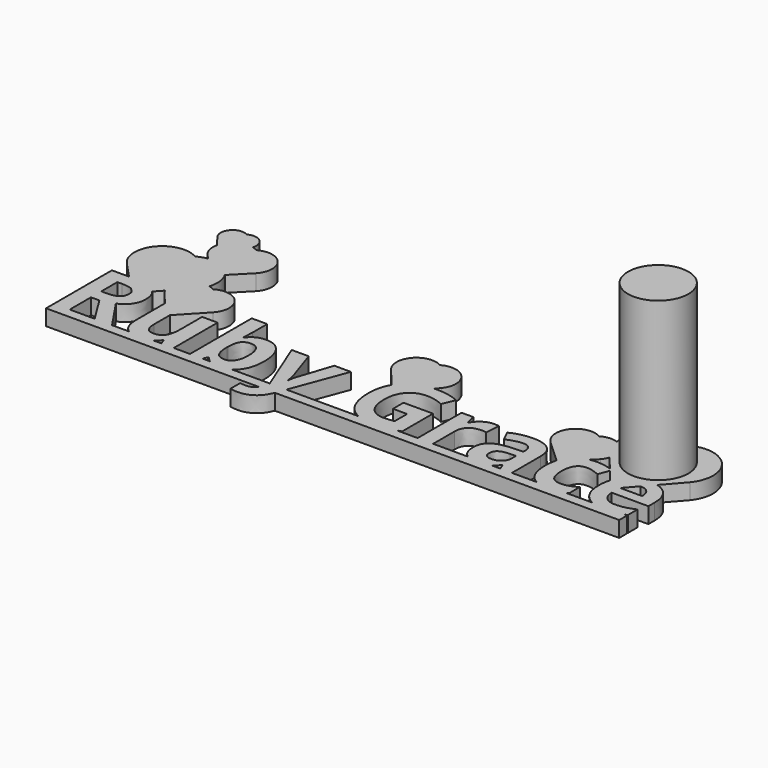
from build123d import *

# Parameters (mm, degrees)
F0_TEXT_SIZE = 13.1857264511
F1_DEPTH     = 2
F2_W         = 72.5544597973
F2_H         = 1.25
F3_DEPTH     = 2
F5_DEPTH     = 2
F6_R         = 3.8242127304
F7_DEPTH     = 20


# Not quite as in the source:
# - a feature names something its author has since deleted; it is built from what else it names
# - Text() gives the source's letters only with a copy of the font that has no kerning and outlines rounded to 1/6400 em; it was checked with that copy


with BuildPart() as f1:
    # F0 (on Top) → F1 (new body)
    with BuildSketch(Plane.XY):
        with Locations((-37.5, -20.9367564448)):
            Text('Ruby Grace', F0_TEXT_SIZE, font='Open Sans', font_style=FontStyle.BOLD, text_align=(TextAlign.LEFT, TextAlign.BOTTOM))
    extrude(amount=F1_DEPTH)

    # F2 (on Top) → F3 (join)
    with BuildSketch(Plane.XY):
        with Locations((-0.0381149905, -21.3117564448)):
            Rectangle(F2_W, F2_H)
    extrude(amount=F3_DEPTH)

    # F4 (on Top) → F5 (join)
    with BuildSketch(Plane.XY):
        with BuildLine():
            ThreePointArc((-22.891365132, -12.3130714182), (-22.7523432909, -9.0480865955), (-25.9622662377, -8.4350224555))
            ThreePointArc((-25.9622662377, -8.4350224555), (-26.2981556025, -8.2731992581), (-26.6543760183, -8.1631291531))
            ThreePointArc((-26.6543760183, -8.1631291531), (-26.7985781504, -8.5405421894), (-26.9853136504, -8.8988223982))
            Line((-26.9853136504, -8.8988223982), (-29.4910691911, -11.6282187871))
            ThreePointArc((-29.4910691911, -11.6282187871), (-29.3216006579, -11.9419906948), (-29.1092122674, -12.2284580847))
            Line((-29.1092122674, -12.2284580847), (-26.104554534, -15.7286860049))
            Line((-26.104554534, -15.7286860049), (-22.891365132, -12.3130714182))
        make_face()
        with BuildLine():
            ThreePointArc((-26.9853136504, -8.8988223982), (-26.7985781504, -8.5405421894), (-26.6543760183, -8.1631291531))
            ThreePointArc((-26.6543760183, -8.1631291531), (-29.1467162118, -9.0164498648), (-29.4910691911, -11.6282187871))
            Line((-29.4910691911, -11.6282187871), (-26.9853136504, -8.8988223982))
        make_face()
        with BuildLine():
            ThreePointArc((-29.4910691911, -11.6282187871), (-29.1467162118, -9.0164498648), (-26.6543760183, -8.1631291531))
            ThreePointArc((-26.6543760183, -8.1631291531), (-26.5125159117, -6.7128085907), (-26.9735699478, -5.3304254314))
            Line((-26.9735699478, -5.3304254314), (-27.8705461931, -6.2434591072))
            Line((-27.8705461931, -6.2434591072), (-30.435701563, -3.633144129))
            ThreePointArc((-30.435701563, -3.633144129), (-31.1099811744, -3.7885760494), (-31.740504166, -4.0736248755))
            ThreePointArc((-31.740504166, -4.0736248755), (-36.233754687, -4.9311026842), (-36.0411839329, -9.5013854919))
            Line((-36.0411839329, -9.5013854919), (-31.7405052483, -14.0784189571))
            Line((-31.7405052483, -14.0784189571), (-29.4910691911, -11.6282187871))
        make_face()
        with BuildLine():
            ThreePointArc((-27.8705461931, -4.3197954554), (-27.3728222762, -4.7814116229), (-26.9735699478, -5.3304254314))
            Line((-26.9735699478, -5.3304254314), (-24.7982677336, -3.1161815346))
            ThreePointArc((-24.7982677336, -3.1161815346), (-24.6612476873, 0.1481262242), (-27.8705463616, 0.7604020253))
            ThreePointArc((-27.8705463616, 0.7604020253), (-28.1874425503, 0.9146740113), (-28.5228848144, 1.0228476104))
            ThreePointArc((-28.5228848144, 1.0228476104), (-28.6581354096, 0.7251189675), (-28.8546919313, 0.4637751287))
            Line((-28.8546919313, 0.4637751287), (-30.8609493077, -1.7959213583))
            Line((-30.8609493077, -1.7959213583), (-31.5607878634, -0.8613195248))
            ThreePointArc((-31.5607878634, -0.8613195248), (-31.5240164461, -2.0926519469), (-30.9036702721, -3.1569368221))
            Line((-30.9036702721, -3.1569368221), (-30.435701563, -3.633144129))
            ThreePointArc((-30.435701563, -3.633144129), (-29.0854748233, -3.7237500646), (-27.8705461931, -4.3197954554))
        make_face()
        with BuildLine():
            Line((-27.8705461931, -6.2434591072), (-26.9735699478, -5.3304254314))
            ThreePointArc((-26.9735699478, -5.3304254314), (-27.3728222762, -4.7814116229), (-27.8705461931, -4.3197954554))
            Line((-27.8705461931, -4.3197954554), (-27.8705461931, -6.2434591072))
        make_face()
        with BuildLine():
            Line((-30.435701563, -3.633144129), (-27.8705461931, -6.2434591072))
            Line((-27.8705461931, -6.2434591072), (-27.8705461931, -4.3197954554))
            ThreePointArc((-27.8705461931, -4.3197954554), (-29.0854748233, -3.7237500646), (-30.435701563, -3.633144129))
        make_face()
        with BuildLine():
            ThreePointArc((-28.8546919313, 0.4637751287), (-28.6581354096, 0.7251189675), (-28.5228848144, 1.0228476104))
            ThreePointArc((-28.5228848144, 1.0228476104), (-30.4382324156, 0.7198861396), (-31.5607878634, -0.8613195248))
            Line((-31.5607878634, -0.8613195248), (-30.8609493077, -1.7959213583))
            Line((-30.8609493077, -1.7959213583), (-28.8546919313, 0.4637751287))
        make_face()
        with BuildLine():
            ThreePointArc((-31.5607878634, -0.8613195248), (-30.4382324156, 0.7198861396), (-28.5228848144, 1.0228476104))
            ThreePointArc((-28.5228848144, 1.0228476104), (-29.002319592, 2.6549750089), (-30.6980615002, 2.7897226685))
            ThreePointArc((-30.6980615002, 2.7897226685), (-32.5699864004, 2.4863172854), (-32.6487473798, 0.5915997956))
            Line((-32.6487473798, 0.5915997956), (-31.5607878634, -0.8613195248))
        make_face()
        with BuildLine():
            ThreePointArc((25.5595961233, -8.9808114981), (24.49969202, -8.8507651041), (23.4822108361, -9.1748651088))
            ThreePointArc((23.4822108361, -9.1748651088), (20.2176636686, -9.8595233663), (20.5393408896, -13.1795457915))
            Line((20.5393408896, -13.1795457915), (23.5436121002, -15.944164712))
            Line((23.5436121002, -15.944164712), (26.6639844478, -12.9268283356))
            ThreePointArc((26.6639844478, -12.9268283356), (26.9346729611, -12.5227898054), (27.1220134693, -12.0739881353))
            Line((27.1220134693, -12.0739881353), (26.4608970103, -11.2691941614))
            ThreePointArc((26.4608970103, -11.2691941614), (25.8299996249, -10.1959947714), (25.5595961233, -8.9808114981))
        make_face()
        with BuildLine():
            ThreePointArc((31.551734789, -5.2660529984), (27.444126715, -5.3304504784), (25.5595961233, -8.9808114981))
            ThreePointArc((25.5595961233, -8.9808114981), (26.9636923968, -10.2127684503), (27.1220134693, -12.0739881353))
            Line((27.1220134693, -12.0739881353), (31.3805904387, -17.2580627952))
            Line((31.3805904387, -17.2580627952), (36.6425725677, -11.2691941614))
            ThreePointArc((36.6425725677, -11.2691941614), (36.6024572806, -6.1430534792), (31.551734789, -5.2660529984))
        make_face()
        with BuildLine():
            ThreePointArc((27.1220134693, -12.0739881353), (26.9636923968, -10.2127684503), (25.5595961233, -8.9808114981))
            ThreePointArc((25.5595961233, -8.9808114981), (25.8299996249, -10.1959947714), (26.4608970103, -11.2691941614))
            Line((26.4608970103, -11.2691941614), (27.1220134693, -12.0739881353))
        make_face()
        with BuildLine():
            ThreePointArc((4.8622423229, -10.8610989956), (4.8371702685, -7.6572610692), (1.6804687113, -7.1091357687))
            ThreePointArc((1.6804687113, -7.1091357687), (-1.476232846, -7.6572610692), (-1.5013049004, -10.8610989956))
            Line((-1.5013049004, -10.8610989956), (1.5735034923, -14.6041418917))
            Line((1.5735034923, -14.6041418917), (4.8622423229, -10.8610989956))
        make_face()
    extrude(amount=F5_DEPTH)

    # F6 (on face) → F7 (join)
    with BuildSketch(Plane.XY.offset(2)):
        with Locations((31.5303290263, -9.8842289299)):
            Circle(F6_R)
    extrude(amount=F7_DEPTH)


solid = f1.part
